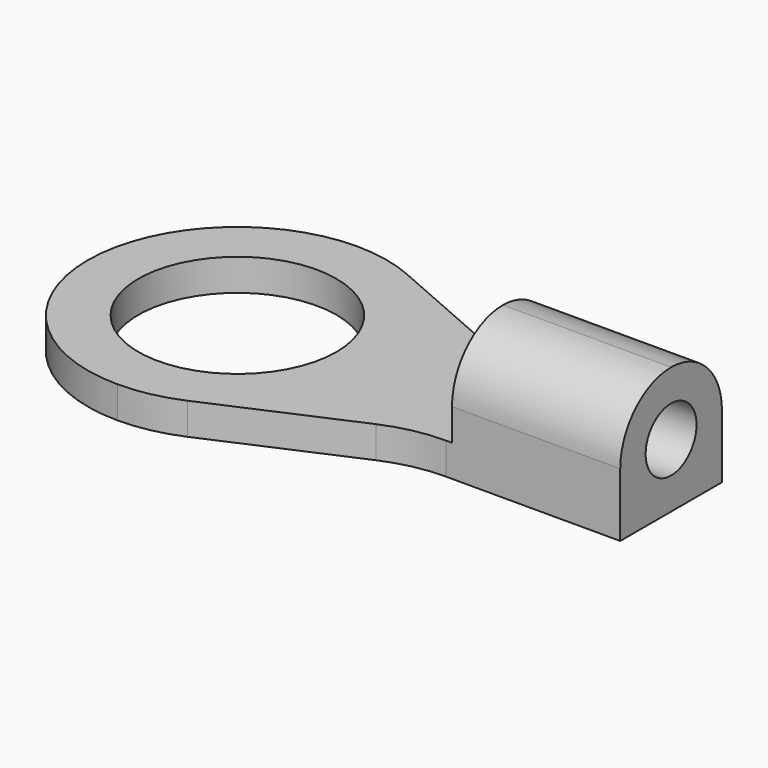
from build123d import *

# Parameters (mm, degrees)
F0_R     = 2.65
F1_DEPTH = 0.85
F2_W     = 4.5
F2_H     = 3.4
F3_DEPTH = 2.55
F4_R     = 1.69999
F5_R     = 0.85
F6_DEPTH = 25


# Not quite as in the source:
# - a fillet or chamfer is up to 0.001 mm smaller than in the source, because OpenCascade refuses the exact size


with BuildPart() as f1:
    # F0 (on Top) → F1 (new body)
    with BuildSketch(Plane.XY):
        with BuildLine():
            Line((10.9356666081, 2.3), (15.6, 2.3))
            Line((15.6, 2.3), (15.6, 5.7))
            Line((15.6, 5.7), (10.9356666081, 5.7))
            ThreePointArc((10.9356666081, 5.7), (10.117660762, 5.7845349656), (9.3342299639, 6.0345667821))
            Line((9.3342299639, 6.0345667821), (5.6014366442, 7.6654332179))
            ThreePointArc((5.6014366442, 7.6654332179), (4.8180058461, 7.9154650344), (4, 8))
            ThreePointArc((4, 8), (1.1715728753, 6.8284271247), (0, 4))
            ThreePointArc((0, 4), (1.1715728753, 1.1715728753), (4, 0))
            ThreePointArc((4, 0), (4.8180058461, 0.0845349656), (5.6014366442, 0.3345667821))
            Line((5.6014366442, 0.3345667821), (9.3342299639, 1.9654332179))
            ThreePointArc((9.3342299639, 1.9654332179), (10.117660762, 2.2154650344), (10.9356666081, 2.3))
        make_face()
        with Locations((4, 4)):
            Circle(F0_R, mode=Mode.SUBTRACT)
    extrude(amount=F1_DEPTH)

    # F2 (on face) → F3 (join)
    with BuildSketch(Plane.XY.offset(0.85)):
        with Locations((13.35, 4)):
            Rectangle(F2_W, F2_H)
    extrude(amount=F3_DEPTH)

    # F4 (radius 1.7 in the source; OpenCascade refuses exactly that, so slightly less here)
    f4_edges = [f1.edges().sort_by_distance(p)[0] for p in [
        (13.35, 5.7, 3.4),
        (13.35, 2.3, 3.4),
    ]]
    fillet(f4_edges, radius=F4_R)

    # F5 (on face) → F6 (cut)
    with BuildSketch(Plane.YZ.offset(15.6)):
        with Locations((4, 1.7)):
            Circle(F5_R)
    extrude(amount=-F6_DEPTH, mode=Mode.SUBTRACT)


solid = f1.part
